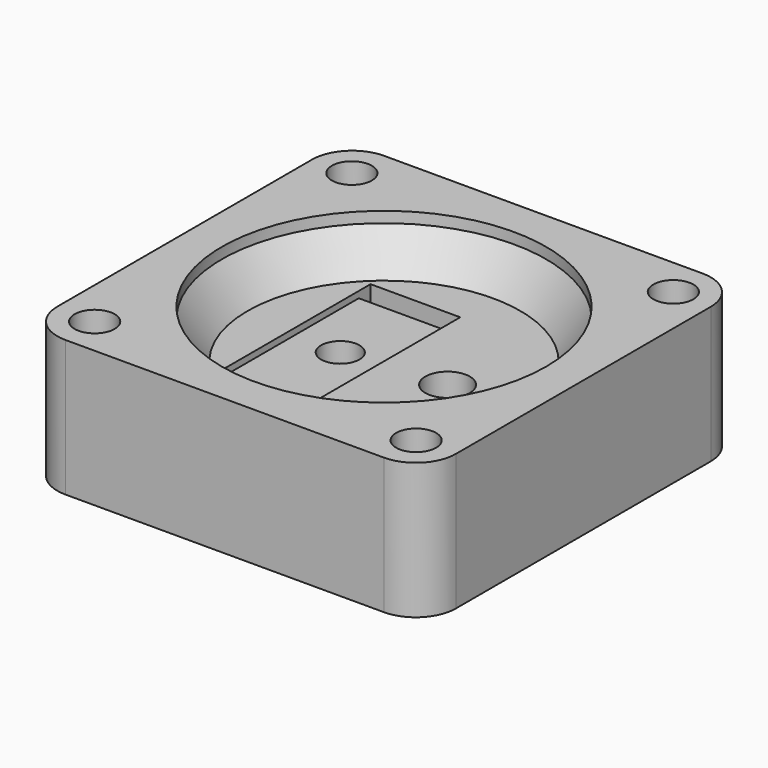
from build123d import *

# Parameters (mm, degrees)
F1_DEPTH        = 10.795
F5_D            = 3.175
F5_COPIES_COUNT = 4
F7_D            = 2.9972
F7_CBORE_D      = 3.5306
F7_CBORE_DEPTH  = 4.6228
F9_D            = 3.048
F10_W           = 7.112
F10_H           = 15.113
F11_DEPTH       = 0.508
F12_W           = 7.112
F12_H           = 1.1684
F13_DEPTH       = 2.159
F15_DEPTH       = 0.8128
F16_W           = 7.112
F16_H           = 15.0114
F17_DEPTH       = 0.508
F18_W           = 7.112
F18_H           = 1.2192
F19_DEPTH       = 2.159
F21_DEPTH       = 0.508


# Not quite as in the source:
# - a pattern or mirror of a feature is missing from the dataset's text; its kind, count and spacing are read off the source's solid


with BuildPart() as f1:
    # F0 (on Top) → F1 (new body)
    with BuildSketch(Plane.XY):
        with BuildLine():
            Line((12.6365, 15.8115), (-12.6365, 15.8115))
            ThreePointArc((-12.6365, 15.8115), (-14.8815640303, 14.8815640303), (-15.8115, 12.6365))
            Line((-15.8115, 12.6365), (-15.8115, -12.6365))
            ThreePointArc((-15.8115, -12.6365), (-14.8815640303, -14.8815640303), (-12.6365, -15.8115))
            Line((-12.6365, -15.8115), (12.6365, -15.8115))
            ThreePointArc((12.6365, -15.8115), (14.8815640303, -14.8815640303), (15.8115, -12.6365))
            Line((15.8115, -12.6365), (15.8115, 12.6365))
            ThreePointArc((15.8115, 12.6365), (14.8815640303, 14.8815640303), (12.6365, 15.8115))
        make_face()
    extrude(amount=F1_DEPTH)

    # F2 (on Front) → F3 (revolve, cut)
    with BuildSketch(Plane.XZ):
        Polygon((0, 10.795), (0, 6.985), (10.8204, 6.985), (12.8651, 9.9314), (12.8651, 10.795), align=None)
    revolve(axis=Axis((0, 0, 1.5018361828), (0, 0, -1)), mode=Mode.SUBTRACT)

    # F5 (through all)
    with Locations(Plane.XY.offset(10.795)):
        with Locations((-12.7519636919, 12.7519636919)):
            f5 = Hole(F5_D / 2)

    # F5_copies: F5 ×4 about axis
    f5_copies_axis = Axis((0, 0, 0), (0, 0, 1))
    for i in range(1, F5_COPIES_COUNT):
        add(f5.rotate(f5_copies_axis, i * 360 / F5_COPIES_COUNT), mode=Mode.SUBTRACT)

    # F7 (through all)
    with Locations(Plane.XY.offset(6.985)):
        with Locations((5.0419, 0)):
            CounterBoreHole(F7_D / 2, F7_CBORE_D / 2, F7_CBORE_DEPTH)

    # F9 (through all)
    with Locations(Plane.XY.offset(6.985)):
        with Locations((-3.4671, 0)):
            Hole(F9_D / 2)

    # F10 (on face) → F11 (cut)
    with BuildSketch(Plane.XY.offset(6.985)):
        with Locations((-3.556, 0)):
            Rectangle(F10_W, F10_H)
    extrude(amount=-F11_DEPTH, mode=Mode.SUBTRACT)

    # F12 (on face) → F13 (cut)
    with BuildSketch(Plane.XY.offset(6.985)):
        with Locations((-3.556, 6.9723)):
            Rectangle(F12_W, F12_H)
    f13 = extrude(amount=-F13_DEPTH, mode=Mode.SUBTRACT)

    # F13_copies: F13 across plane
    add(f13.mirror(Plane(origin=(0, 0, 0), x_dir=(0, 0, -1), z_dir=(0, -1, 0))), mode=Mode.SUBTRACT)

    # F14 (on face) → F15 (cut)
    with BuildSketch(Plane(origin=(0, 0, 0), x_dir=(1, 0, 0), z_dir=(0, 0, -1))):
        with BuildLine():
            ThreePointArc((1.4097, -12.8524), (12.9413, 0), (1.4097, 12.8524))
            Line((1.4097, 12.8524), (1.4097, -12.8524))
        make_face()
    extrude(amount=-F15_DEPTH, mode=Mode.SUBTRACT)

    # F16 (on face) → F17 (cut)
    with BuildSketch(Plane(origin=(0, 0, 0.8128), x_dir=(1, 0, 0), z_dir=(0, 0, -1))):
        with Locations((4.9657, 0)):
            Rectangle(F16_W, F16_H)
    extrude(amount=-F17_DEPTH, mode=Mode.SUBTRACT)

    # F18 (on face) → F19 (cut)
    with BuildSketch(Plane(origin=(0, 0, 0.8128), x_dir=(1, 0, 0), z_dir=(0, 0, -1))):
        with Locations((4.9657, 6.8961)):
            Rectangle(F18_W, F18_H)
    f19 = extrude(amount=-F19_DEPTH, mode=Mode.SUBTRACT)

    # F19_copies: F19 across plane
    add(f19.mirror(Plane.ZX), mode=Mode.SUBTRACT)

    # F20 (on face) → F21 (cut, through all)
    with BuildSketch(Plane(origin=(0, 0, 0.8128), x_dir=(1, 0, 0), z_dir=(0, 0, -1))):
        with BuildLine():
            Line((11.9371615818, 1.3470384182), (8.5217, 4.7625))
            Line((8.5217, 4.7625), (8.5217, -4.7625))
            Line((8.5217, -4.7625), (11.9371615818, -1.3470384182))
            ThreePointArc((11.9371615818, -1.3470384182), (12.4951231637, 0), (11.9371615818, 1.3470384182))
        make_face()
    extrude(amount=-F21_DEPTH, mode=Mode.SUBTRACT)


solid = f1.part
